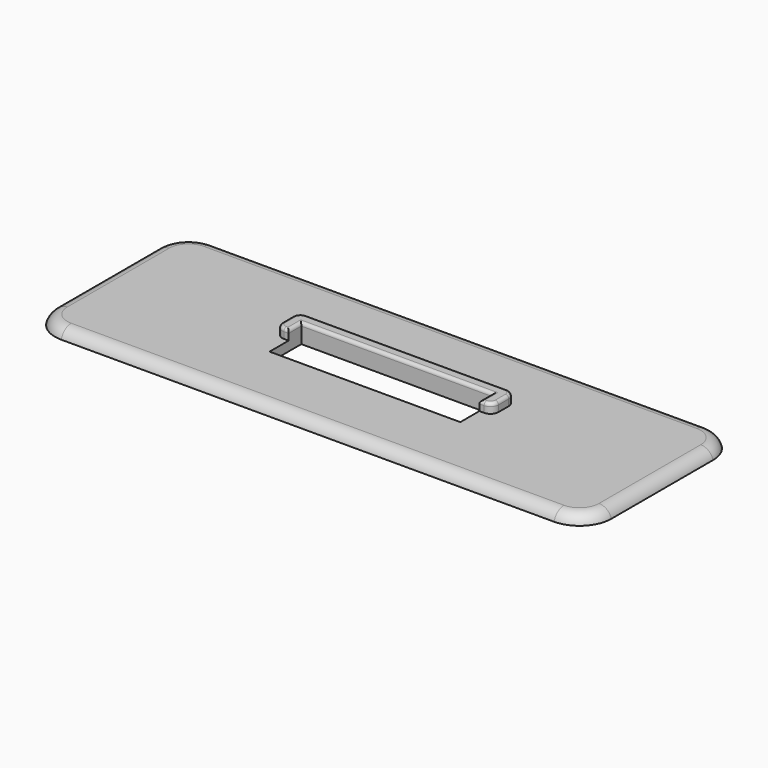
from build123d import *

# Parameters (mm, degrees)
F0_W         = 35
F0_H         = 12
F0_W_2       = 12
F0_H_2       = 2
F1_DEPTH     = 0.6
F3_DEPTH     = 0.6
F4_R         = 2
F5_R         = 0.5
F6_SIZE      = 0.5
F7_T1_DEPTH  = 8
F7_T3_DEPTH  = 31
F7_T6_ANGLE  = 90
F7_T8_ANGLE  = 90
F7_T10_ANGLE = 90
F7_T12_ANGLE = 90
F8_R         = 0.2


# Not quite as in the source:
# - a fillet or chamfer that OpenCascade refuses, or shapes differently, is made with other operations: its cross-section is extruded or revolved along the edge and cut away or added


with BuildPart() as f1:
    # F0 (on Top) → F1 (new body)
    with BuildSketch(Plane.XY):
        Rectangle(F0_W, F0_H)
        Rectangle(F0_W_2, F0_H_2, mode=Mode.SUBTRACT)
    extrude(amount=F1_DEPTH)

    # F2 (on face) → F3 (join)
    with BuildSketch(Plane.XY.offset(0.6)):
        Polygon((-6.8, 0), (-6, 0), (-6, 1), (6, 1), (6, 0), (6.8, 0), (6.8, 1.8), (-6.8, 1.8), align=None)
    extrude(amount=F3_DEPTH)

    # F4
    f4_edges = [f1.edges().sort_by_distance(p)[0] for p in [
        (-17.5, -6, 0.3),
        (-17.5, 6, 0.3),
        (17.5, 6, 0.3),
        (17.5, -6, 0.3),
    ]]
    fillet(f4_edges, radius=F4_R)

    # F5
    f5_edges = [f1.edges().sort_by_distance(p)[0] for p in [
        (6.8, 1.8, 0.9),
        (6.8, 0, 0.9),
        (-6.8, 1.8, 0.9),
        (-6.8, 0, 0.9),
    ]]
    fillet(f5_edges, radius=F5_R)

    # F6
    f6_edges = [f1.edges().sort_by_distance(p)[0] for p in [
        (0, -1, 0.6),
    ]]
    chamfer(f6_edges, length=F6_SIZE)

    # F7: fillet of radius 0.8 on 8 edges, made by hand

    # F7_s2 → F7_t1 (cut)
    with BuildSketch(Plane.XZ.offset(-4)):
        with BuildLine():
            ThreePointArc((16.7254033308, 0.6), (17.2153012793, 0.432455532), (17.5, 0))
            Line((17.5, 0), (17.5, 0.6))
            Line((17.5, 0.6), (16.7254033308, 0.6))
        make_face()
        with BuildLine():
            ThreePointArc((-16.7254033308, 0.6), (-17.2153012793, 0.432455532), (-17.5, 0))
            Line((-17.5, 0), (-17.5, 0.6))
            Line((-17.5, 0.6), (-16.7254033308, 0.6))
        make_face()
    extrude(amount=F7_T1_DEPTH, mode=Mode.SUBTRACT)

    # F7_s4 → F7_t3 (cut)
    with BuildSketch(Plane.YZ.offset(-15.5)):
        with BuildLine():
            ThreePointArc((5.2254033308, 0.6), (5.7153012793, 0.432455532), (6, 0))
            Line((6, 0), (6, 0.6))
            Line((6, 0.6), (5.2254033308, 0.6))
        make_face()
        with BuildLine():
            ThreePointArc((-5.2254033308, 0.6), (-5.7153012793, 0.432455532), (-6, 0))
            Line((-6, 0), (-6, 0.6))
            Line((-6, 0.6), (-5.2254033308, 0.6))
        make_face()
    extrude(amount=F7_T3_DEPTH, mode=Mode.SUBTRACT)

    # F7_s5 → F7_t6 (revolve, cut)
    with BuildSketch(Plane.YZ.offset(15.5)):
        with BuildLine():
            ThreePointArc((5.2254033308, 0.6), (5.7153012793, 0.432455532), (6, 0))
            Line((6, 0), (6, 0.6))
            Line((6, 0.6), (5.2254033308, 0.6))
        make_face()
    revolve(axis=Axis((15.5, 4, 0.6), (0, 0, -1)), revolution_arc=F7_T6_ANGLE, mode=Mode.SUBTRACT)

    # F7_s7 → F7_t8 (revolve, cut)
    with BuildSketch(Plane.YZ.offset(15.5)):
        with BuildLine():
            ThreePointArc((-5.2254033308, 0.6), (-5.7153012793, 0.432455532), (-6, 0))
            Line((-6, 0), (-6, 0.6))
            Line((-6, 0.6), (-5.2254033308, 0.6))
        make_face()
    revolve(axis=Axis((15.5, -4, 0.6), (0, 0, 1)), revolution_arc=F7_T8_ANGLE, mode=Mode.SUBTRACT)

    # F7_s9 → F7_t10 (revolve, cut)
    with BuildSketch(Plane.YZ.offset(-15.5)):
        with BuildLine():
            ThreePointArc((-5.2254033308, 0.6), (-5.7153012793, 0.432455532), (-6, 0))
            Line((-6, 0), (-6, 0.6))
            Line((-6, 0.6), (-5.2254033308, 0.6))
        make_face()
    revolve(axis=Axis((-15.5, -4, 0.6), (0, 0, -1)), revolution_arc=F7_T10_ANGLE, mode=Mode.SUBTRACT)

    # F7_s11 → F7_t12 (revolve, cut)
    with BuildSketch(Plane.YZ.offset(-15.5)):
        with BuildLine():
            ThreePointArc((5.2254033308, 0.6), (5.7153012793, 0.432455532), (6, 0))
            Line((6, 0), (6, 0.6))
            Line((6, 0.6), (5.2254033308, 0.6))
        make_face()
    revolve(axis=Axis((-15.5, 4, 0.6), (0, 0, 1)), revolution_arc=F7_T12_ANGLE, mode=Mode.SUBTRACT)

    # F8
    f8_edges = [f1.edges().sort_by_distance(p)[0] for p in [
        (6.15, 0, 1.2),
        (6.653553, 0.146447, 1.2),
        (6.8, 0.9, 1.2),
        (6.653553, 1.653553, 1.2),
        (0, 1.8, 1.2),
        (-6.653553, 1.653553, 1.2),
        (-6.8, 0.9, 1.2),
        (-6.653553, 0.146447, 1.2),
        (-6.15, 0, 1.2),
        (-6, 0.5, 1.2),
        (0, 1, 1.2),
        (6, 0.5, 1.2),
    ]]
    fillet(f8_edges, radius=F8_R)


solid = f1.part
